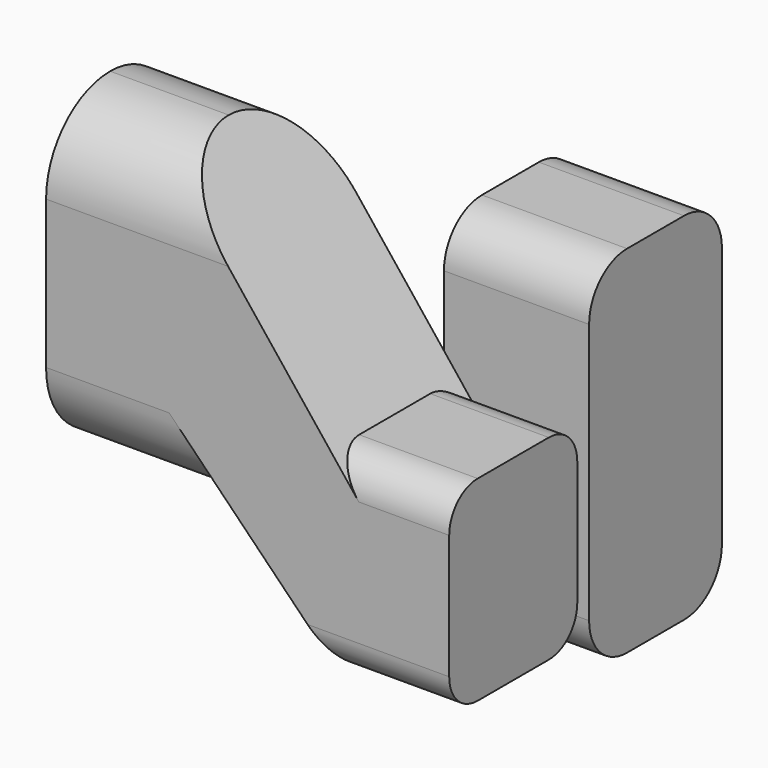
from build123d import *

# Parameters (mm, degrees)
F1_DEPTH = 13.5
F2_R     = 6.74999
F3_R     = 3
F4_W     = 12.2435482951
F4_H     = 30
F5_DEPTH = 14
F6_R     = 4


# Not quite as in the source:
# - a fillet or chamfer is up to 0.001 mm smaller than in the source, because OpenCascade refuses the exact size


with BuildPart() as f1:
    # F0 (on Front) → F1 (new body)
    with BuildSketch(Plane.XZ):
        Polygon((0, 26), (0, 0), (17, 0), (25, -8.16), (34, -8.16), (34, 8.34), (24, 8.34), (10, 26), align=None)
    extrude(amount=F1_DEPTH)

    # F2 (radius 6.75 in the source; OpenCascade refuses exactly that, so slightly less here)
    f2_edges = [f1.edges().sort_by_distance(p)[0] for p in [
        (5, 0, 26),
        (5, -13.5, 26),
        (8.5, 0, 0),
        (8.5, -13.5, 0),
    ]]
    fillet(f2_edges, radius=F2_R)

    # F3
    f3_edges = [f1.edges().sort_by_distance(p)[0] for p in [
        (29, -13.5, 8.34),
        (29, 0, 8.34),
        (29.5, 0, -8.16),
        (29.5, -13.5, -8.16),
    ]]
    fillet(f3_edges, radius=F3_R)

    # F4 (on face) → F5 (join)
    with BuildSketch(Plane(origin=(0, 0, 0), x_dir=(-1, 0, 0), z_dir=(0, 1, 0))):
        with Locations((-28.8782258524, 4.84)):
            Rectangle(F4_W, F4_H)
    extrude(amount=F5_DEPTH)

    # F6
    f6_edges = [f1.edges().sort_by_distance(p)[0] for p in [
        (28.878226, 14, 19.84),
        (28.878226, 0, 19.84),
        (28.878226, 14, -10.16),
        (28.878226, 0, -10.16),
    ]]
    fillet(f6_edges, radius=F6_R)


solid = f1.part
